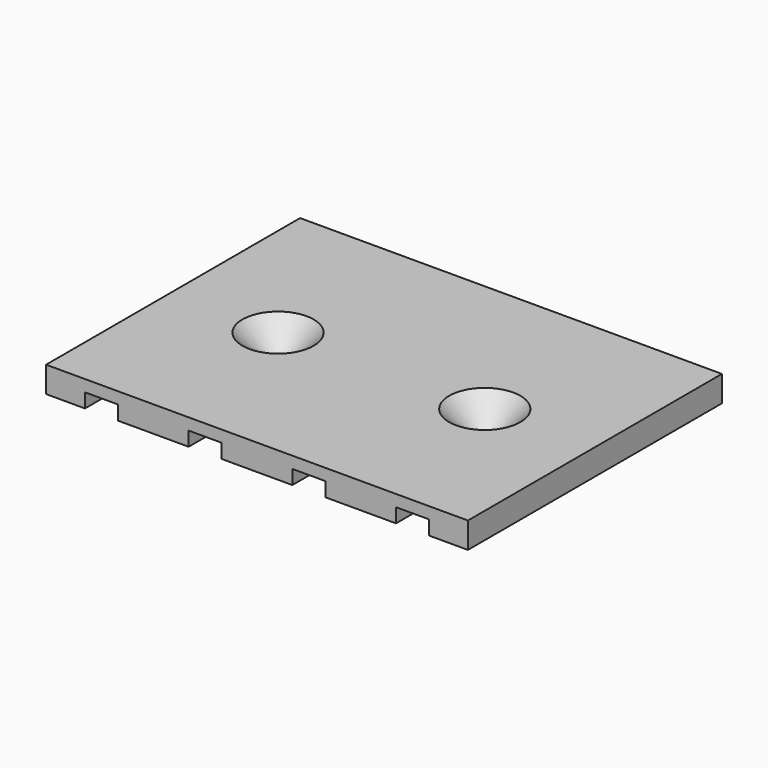
from build123d import *

# Parameters (mm, degrees)
F1_DEPTH      = 49
F2_R          = 1.5
F3_DEPTH      = 25
F3_DEPTH_BACK = 25
F4_DEPTH      = 12.4
F5_SIZE       = 3.99999


# Not quite as in the source:
# - a fillet or chamfer is up to 0.001 mm smaller than in the source, because OpenCascade refuses the exact size
# - a feature names something its author has since deleted; it is built from what else it names


with BuildPart() as f1:
    # F0 (on Front) → F1 (new body)
    with BuildSketch(Plane.XZ):
        Polygon((-16.275, 4), (-32.55, 4), (-32.55, 0), (-26.55, 0), (-26.55, 2.2), (-21.45, 2.2), (-21.45, 0), (-16.275, 0), align=None)
        Polygon((0, 4), (-16.275, 4), (-16.275, 0), (-10.55, 0), (-10.55, 2.2), (-5.45, 2.2), (-5.45, 0), (0, 0), align=None)
        Polygon((16.275, 4), (0, 4), (0, 0), (5.45, 0), (5.45, 2.2), (10.55, 2.2), (10.55, 0), (16.275, 0), align=None)
        Polygon((32.55, 4), (16.275, 4), (16.275, 0), (21.45, 0), (21.45, 2.2), (26.55, 2.2), (26.55, 0), (32.55, 0), align=None)
    extrude(amount=F1_DEPTH)

    # F2 (on Top) → F3 (cut, two sides)
    with BuildSketch(Plane.XY) as f3_sk:
        with Locations((-15.95, -25)):
            Circle(F2_R)
    extrude(amount=-F3_DEPTH, mode=Mode.SUBTRACT)
    extrude(f3_sk.sketch, amount=F3_DEPTH_BACK, mode=Mode.SUBTRACT)

    # F2 (on Top) → F4 (cut)
    with BuildSketch(Plane.XY):
        with Locations((-15.95, -25)):
            Circle(F2_R)
        with Locations((15.95, -25)):
            Circle(F2_R)
    extrude(amount=F4_DEPTH, mode=Mode.SUBTRACT)

    # F5 (size 4 in the source; OpenCascade refuses exactly that, so slightly less here)
    f5_edges = [f1.edges().sort_by_distance(p)[0] for p in [
        (14.45, -25, 4),
        (-17.45, -25, 4),
    ]]
    chamfer(f5_edges, length=F5_SIZE)


solid = f1.part
